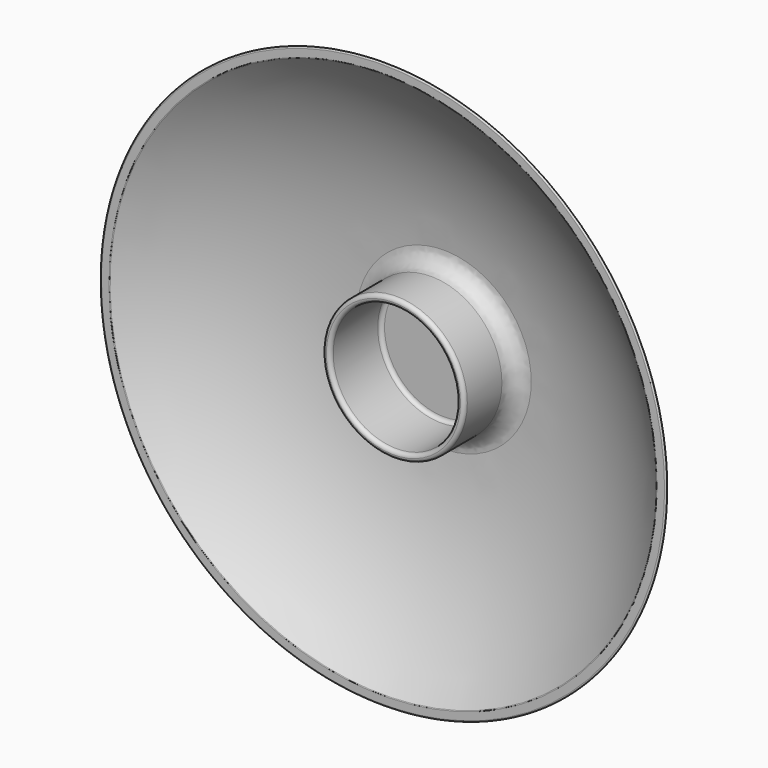
from build123d import *

# Parameters (mm, degrees)
F2_R = 5
F3_R = 1.2
F4_R = 1.19999
F5_R = 0.4


# Not quite as in the source:
# - a fillet or chamfer is up to 0.001 mm smaller than in the source, because OpenCascade refuses the exact size


with BuildPart() as f1:
    # F0 (on Top) → F1 (revolve)
    with BuildSketch(Plane.XY):
        with BuildLine():
            Line((22.4, 32.7261249118), (0, 32.7261249118))
            Line((0, 32.7261249118), (0, 30.3261249118))
            Line((0, 30.3261249118), (20, 30.3261249118))
            Line((20, 30.3261249118), (20, 10.3261249118))
            Line((20, 10.3261249118), (22.4, 10.3261249118))
            Line((22.4, 10.3261249118), (22.4, 30.3261249118))
            ThreePointArc((22.4, 30.3261249118), (56.6048812575, 24.0969709185), (86.417783153, 6.2093455344))
            Line((86.417783153, 6.2093455344), (90, 6.2093455344))
            ThreePointArc((90, 6.2093455344), (58.7073669816, 25.8598390885), (22.4, 32.7261249118))
        make_face()
    revolve(axis=Axis((0, 32.0515017956, 0), (0, -1, 0)))

    # F2
    f2_edges = [f1.edges().sort_by_distance(p)[0] for p in [
        (-22.4, 30.326125, 0),
    ]]
    fillet(f2_edges, radius=F2_R)

    # F3
    f3_edges = [f1.edges().sort_by_distance(p)[0] for p in [
        (-20, 30.326125, 0),
    ]]
    fillet(f3_edges, radius=F3_R)

    # F4 (radius 1.2 in the source; OpenCascade refuses exactly that, so slightly less here)
    f4_edges = [f1.edges().sort_by_distance(p)[0] for p in [
        (-20, 10.326125, 0),
        (-22.4, 10.326125, 0),
    ]]
    fillet(f4_edges, radius=F4_R)

    # F5
    f5_edges = [f1.edges().sort_by_distance(p)[0] for p in [
        (-90, 6.209346, 0),
        (-86.417783, 6.209346, 0),
    ]]
    fillet(f5_edges, radius=F5_R)


solid = f1.part
